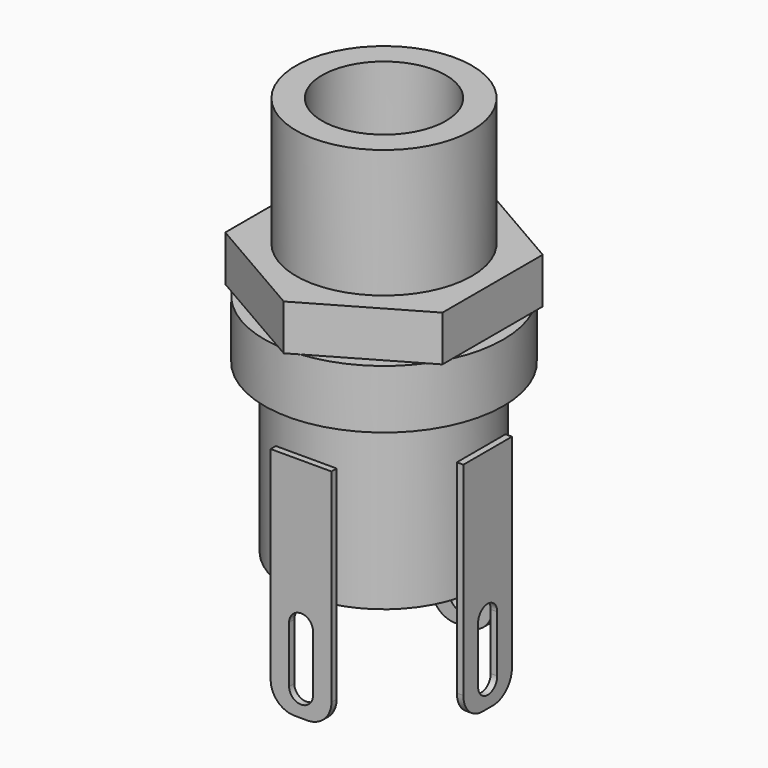
from build123d import *

# Parameters (mm, degrees)
F0_R      = 4.05
F0_R_2    = 2.85
F1_DEPTH  = 8
F3_DEPTH  = 2.1
F4_R      = 5.5
F5_DEPTH  = 2.7
F6_R      = 4.475
F7_DEPTH  = 7.7
F10_DEPTH = 0.3
F11_COUNT = 3
F11_ANGLE = 180


with BuildPart() as f1:
    # F0 (on Top) → F1 (new body)
    with BuildSketch(Plane.XY):
        Circle(F0_R)
        Circle(F0_R_2, mode=Mode.SUBTRACT)
    extrude(amount=F1_DEPTH)

    # F2 (on face) → F3 (join)
    with BuildSketch(Plane(origin=(0, 0, 0), x_dir=(1, 0, 0), z_dir=(0, 0, -1))):
        Polygon((5, -2.8867513459), (5, 2.8867513459), (0, 5.7735026919), (-5, 2.8867513459), (-5, -2.8867513459), (0, -5.7735026919), align=None)
    extrude(amount=-F3_DEPTH)

    # F4 (on face) → F5 (join)
    with BuildSketch(Plane(origin=(0, 0, 0), x_dir=(1, 0, 0), z_dir=(0, 0, -1))):
        Circle(F4_R)
    extrude(amount=F5_DEPTH)

    # F6 (on face) → F7 (join)
    with BuildSketch(Plane(origin=(0, 0, -2.7), x_dir=(1, 0, 0), z_dir=(0, 0, -1))):
        Circle(F6_R)
    extrude(amount=F7_DEPTH)


with BuildPart() as f10:
    # F9 (on offset) → F10 (new body)
    with BuildSketch(Plane.XZ.offset(4.475)):
        with BuildLine():
            ThreePointArc((-1.4, -14.1), (-1.0778174593, -14.8778174593), (-0.3, -15.2))
            Line((-0.3, -15.2), (0.3, -15.2))
            ThreePointArc((0.3, -15.2), (1.0778174593, -14.8778174593), (1.4, -14.1))
            Line((1.4, -14.1), (1.4, -4.7437562607))
            Line((1.4, -4.7437562607), (-1.4, -4.7437562607))
            Line((-1.4, -4.7437562607), (-1.4, -14.1))
        make_face()
        with BuildLine():
            Line((0.55, -11.5), (0.55, -14.1))
            ThreePointArc((0.55, -14.1), (0, -14.65), (-0.55, -14.1))
            Line((-0.55, -14.1), (-0.55, -11.5))
            ThreePointArc((-0.55, -11.5), (0, -10.95), (0.55, -11.5))
        make_face(mode=Mode.SUBTRACT)
    extrude(amount=F10_DEPTH)


with BuildPart() as f11_1:
    # F11: instance of F10
    add(f10.part.rotate(Axis((0, 0, 8), (0, 0, 1)), 1 * F11_ANGLE / (F11_COUNT - 1)))


with BuildPart() as f11_2:
    # F11: instance of F10
    add(f10.part.rotate(Axis((0, 0, 8), (0, 0, 1)), 2 * F11_ANGLE / (F11_COUNT - 1)))


solid = Compound([f1.part, f10.part, f11_1.part, f11_2.part])
